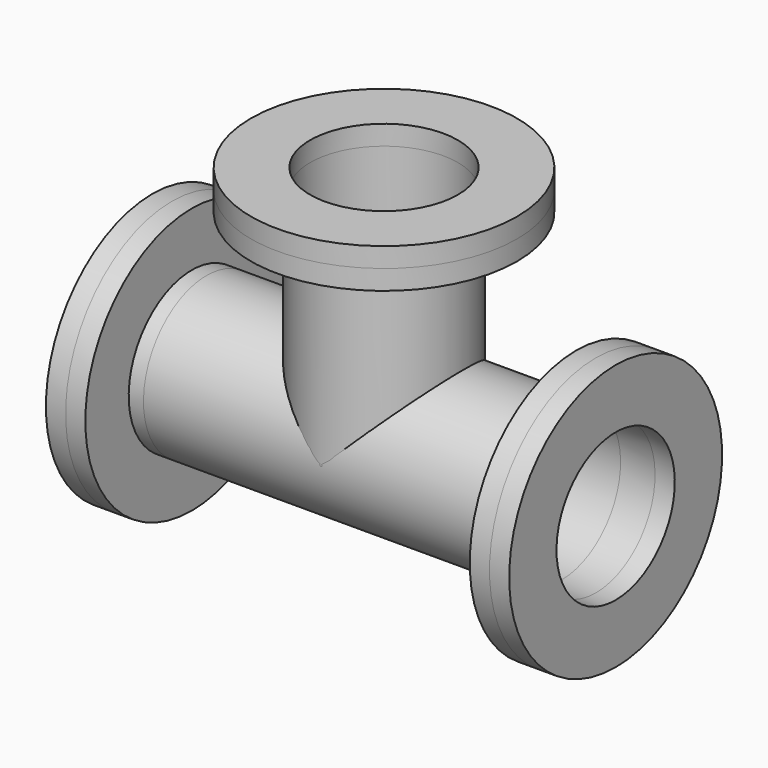
from build123d import *

# Parameters (mm, degrees)
F0_R      = 101.6
F0_R_2    = 95.25
F1_DEPTH  = 19.05
F2_R      = 171.45
F2_R_2    = 101.6
F2_R_3    = 95.25
F3_DEPTH  = 25.4
F9_ANGLE  = 90
F11_DEPTH = 457.2
F12_REACH = 687.4191958742
F13_DEPTH = 25.4
F14_DEPTH = 25.4
F15_DEPTH = 25.4


with BuildPart() as f1:
    # F0 (on Top) → F1 (new body)
    with BuildSketch(Plane.XY):
        Circle(F0_R)
        Circle(F0_R_2, mode=Mode.SUBTRACT)
    extrude(amount=F1_DEPTH)

    # F2 (on face) → F3 (join)
    with BuildSketch(Plane.XY.offset(19.05)):
        Circle(F2_R)
        Circle(F2_R_2, mode=Mode.SUBTRACT)
        Circle(F2_R_2)
        Circle(F2_R_3, mode=Mode.SUBTRACT)
    extrude(amount=F3_DEPTH)


with BuildPart() as f7_1:
    # F7: copy of F1
    add(f1.part.moved(Location((228.6, 0, -228.6))))


with BuildPart() as f7_1_1:
    # F9: moved
    add(f7_1.part.rotate(Axis((228.6, 122.1911609173, -228.6), (0, 1, 0)), F9_ANGLE))


with BuildPart() as f10_1:
    # F10: instance of F7_1
    add(f7_1_1.part.mirror(Plane.YZ))


with BuildPart() as f7_1_2:
    add(f7_1_1.part)

    # F11 (add, through all): a face of the model
    f11_faces = [f7_1_2.faces().sort_by_distance(p)[0] for p in [
        (228.6, 0, -129.8736819587),
    ]]

    add(f10_1.part)  # F11 merges F10_1
    extrude(f11_faces, amount=F11_DEPTH)


with BuildPart() as f1_1:
    add(f1.part)

    f12_end = f7_1_2.part.faces().sort_by_distance((0, 0, -127))[0]
    # F0 (on Top) → F12 (join, up to a face of F7_1 that its end follows)
    with BuildSketch(Plane.XY):
        Circle(F0_R)
        Circle(F0_R_2, mode=Mode.SUBTRACT)
    f12_long = extrude(amount=-F12_REACH, mode=Mode.PRIVATE)
    add(split(f12_long, bisect_by=f12_end, keep=Keep.ALL, mode=Mode.PRIVATE).solids().sort_by_distance((-98.7263180413, 0, 0))[0])


with BuildPart() as f13:
    # F13 (new): a face of the model
    f13_faces = [f1_1.part.faces().sort_by_distance(p)[0] for p in [
        (-166.6006616946, 0, 44.45),
    ]]
    extrude(f13_faces, amount=F13_DEPTH)


with BuildPart() as f14:
    # F14 (new): a face of the model
    f14_faces = [f7_1_2.part.faces().sort_by_distance(p)[0] for p in [
        (273.05, 0, -61.9993383054),
    ]]
    extrude(f14_faces, amount=F14_DEPTH)


with BuildPart() as f15:
    # F15 (new): a face of the model
    f15_faces = [f7_1_2.part.faces().sort_by_distance(p)[0] for p in [
        (-273.05, 0, -61.9993383054),
    ]]
    extrude(f15_faces, amount=F15_DEPTH)


solid = Compound([f7_1_2.part, f1_1.part, f13.part, f14.part, f15.part])
